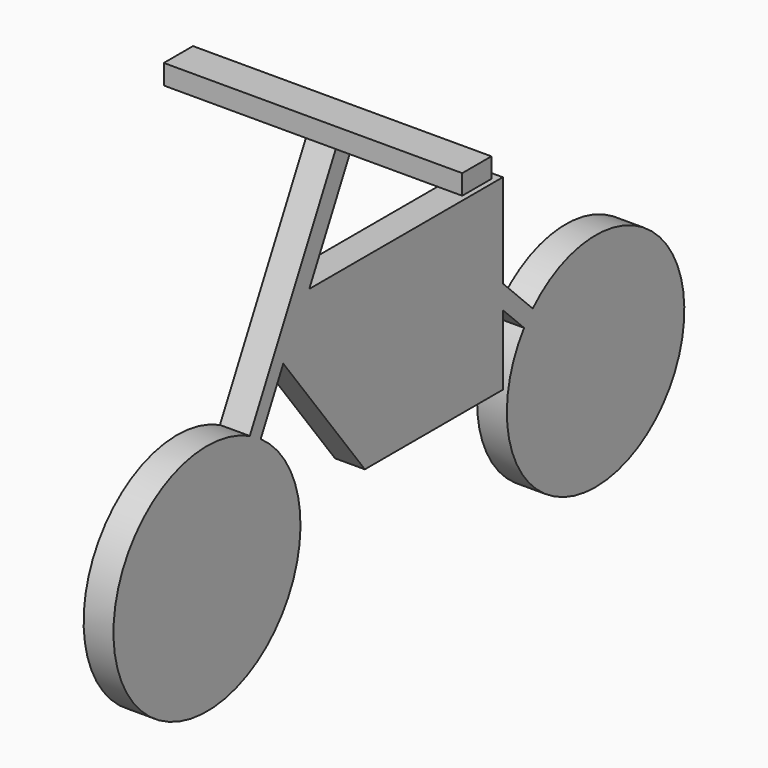
from build123d import *

# Parameters (mm, degrees)
F1_DEPTH = 45
F2_DEPTH = 450


# Not quite as in the source:
# - a feature names something its author has since deleted; it is built from what else it names


with BuildPart() as f1:
    # F0 (on Right) → F1 (new body, symmetric)
    with BuildSketch(Plane.YZ):
        with BuildLine():
            ThreePointArc((161.2936216865, 313.43359361), (-300.9254489442, -183.5759357262), (352.5, 0))
            ThreePointArc((352.5, 0), (312.7518796274, 162.6115364588), (202.4715643149, 288.5507158956))
            ThreePointArc((202.4715643149, 288.5507158956), (182.3076165098, 301.6955136599), (161.2936216865, 313.43359361))
        make_face()
        with BuildLine():
            ThreePointArc((161.2936216865, 313.43359361), (182.3076165098, 301.6955136599), (202.4715643149, 288.5507158956))
            Line((202.4715643149, 288.5507158956), (287.6534110047, 454.0802144534))
            Line((287.6534110047, 454.0802144534), (255.5, 496.5))
            Line((255.5, 496.5), (161.2936216865, 313.43359361))
        make_face()
        Polygon((255.5, 496.5), (287.6534110047, 454.0802144534), (595.193856999, 48.3441087551), (1115.193856999, 48.3441087551), (1115.193856999, 259.8511291536), (1115.193856999, 330.4220543775), (1115.193856999, 612.5), (385.6319234642, 612.5), (315.193856999, 612.5), align=None)
        Polygon((495.5619335347, 963), (315.193856999, 612.5), (385.6319234642, 612.5), (566, 963), align=None)
        Polygon((456, 963), (495.5619335347, 963), (566, 963), (566, 1023), (456, 1023), align=None)
        with BuildLine():
            Line((1115.193856999, 330.4220543775), (1115.193856999, 259.8511291536))
            Line((1115.193856999, 259.8511291536), (1195.3817888304, 179.9804793552))
            ThreePointArc((1195.3817888304, 179.9804793552), (1210.9786128275, 199.6313048689), (1228.0043825139, 218.0578897059))
            Line((1228.0043825139, 218.0578897059), (1115.193856999, 330.4220543775))
        make_face()
        with BuildLine():
            ThreePointArc((1228.0043825139, 218.0578897059), (1210.9786128275, 199.6313048689), (1195.3817888304, 179.9804793552))
            ThreePointArc((1195.3817888304, 179.9804793552), (1360.8295666617, -335.8659636043), (1799.5, -18))
            ThreePointArc((1799.5, -18), (1592.7012450035, 291.1644255482), (1228.0043825139, 218.0578897059))
        make_face()
    extrude(amount=F1_DEPTH, both=True)

    # F0 (on Right) → F2 (join, symmetric)
    with BuildSketch(Plane.YZ):
        Polygon((456, 963), (495.5619335347, 963), (566, 963), (566, 1023), (456, 1023), align=None)
    extrude(amount=F2_DEPTH, both=True)


solid = f1.part
